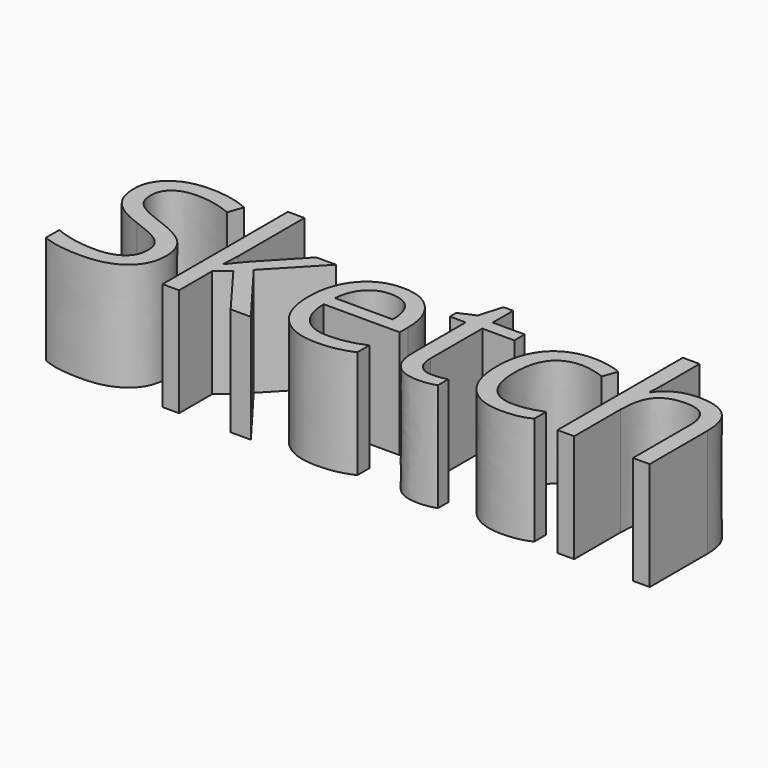
from build123d import *

# Parameters (mm, degrees)
F0_TEXT_SIZE = 580.6603051487
F1_DEPTH     = 304.8


# Not quite as in the source:
# - Text() gives the source's letters only with a copy of the font that has no kerning and outlines rounded to 1/6400 em; it was checked with that copy


with BuildPart() as f1:
    # F0 (on Top) → F1 (new body)
    with BuildSketch(Plane.XY):
        with Locations((228.1275769986, -418.0754197071)):
            Text('Sketch', F0_TEXT_SIZE, font='Open Sans', text_align=(TextAlign.LEFT, TextAlign.BOTTOM))
    extrude(amount=F1_DEPTH)


solid = f1.part
